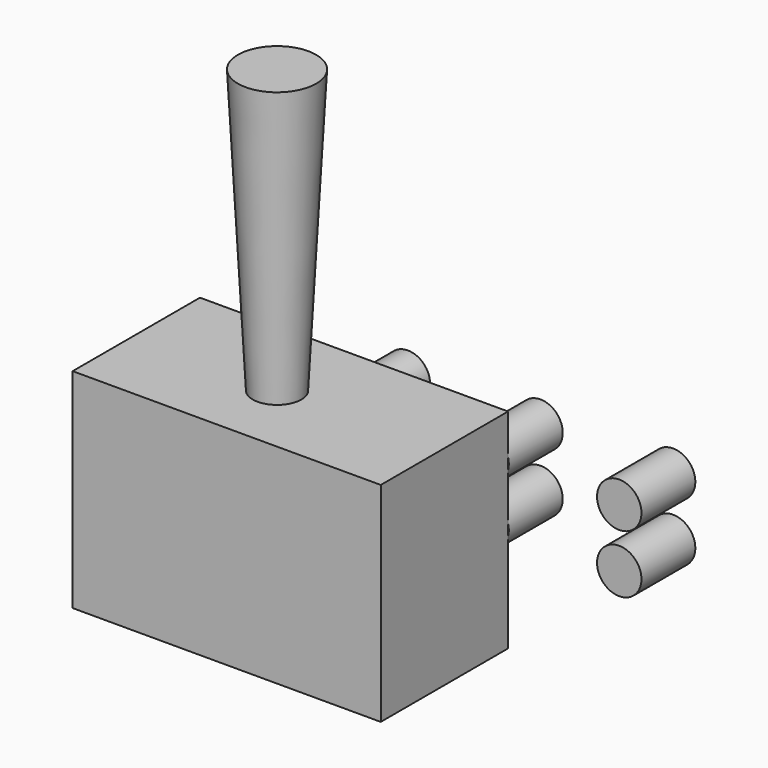
from build123d import *

# Parameters (mm, degrees)
F0_W     = 58.0838136375
F0_H     = 39.3294803798
F1_DEPTH = 30
F2_R     = 4.1888514279
F3_DEPTH = 12.7
F4_R     = 3.5500300139
F5_DEPTH = 73
F5_TAPER = -3


with BuildPart() as f1:
    # F0 (on Front) → F1 (new body)
    with BuildSketch(Plane.XZ):
        Rectangle(F0_W, F0_H)
    extrude(amount=F1_DEPTH)


with BuildPart() as f3:
    # F2 (on Front) → F3 (new body)
    with BuildSketch(Plane.XZ):
        Circle(F2_R)
    extrude(amount=-F3_DEPTH)


with BuildPart() as f3b:
    # F2 (on Front) → F3, piece 2 (new body)
    with BuildSketch(Plane.XZ):
        with Locations((0, 11)):
            Circle(F2_R)
    extrude(amount=-F3_DEPTH)


with BuildPart() as f3c:
    # F2 (on Front) → F3, piece 3 (new body)
    with BuildSketch(Plane.XZ):
        with Locations((25, 0)):
            Circle(F2_R)
    extrude(amount=-F3_DEPTH)


with BuildPart() as f3d:
    # F2 (on Front) → F3, piece 4 (new body)
    with BuildSketch(Plane.XZ):
        with Locations((25, 11)):
            Circle(F2_R)
    extrude(amount=-F3_DEPTH)


with BuildPart() as f3e:
    # F2 (on Front) → F3, piece 5 (new body)
    with BuildSketch(Plane.XZ):
        with Locations((50, 0)):
            Circle(F2_R)
    extrude(amount=-F3_DEPTH)


with BuildPart() as f3f:
    # F2 (on Front) → F3, piece 6 (new body)
    with BuildSketch(Plane.XZ):
        with Locations((50, 11)):
            Circle(F2_R)
    extrude(amount=-F3_DEPTH)


with BuildPart() as f5:
    # F4 (on Top) → F5 (new body)
    with BuildSketch(Plane.XY):
        with Locations((-1.6740621068, -16.0430576652)):
            Circle(F4_R)
    extrude(amount=F5_DEPTH, taper=F5_TAPER)


with BuildPart() as f1_1:
    add(f1.part)

    # F6: cut F5
    add(f5.part, mode=Mode.SUBTRACT)


solid = Compound([f3.part, f3b.part, f3c.part, f3d.part, f3e.part, f3f.part, f5.part, f1_1.part])
